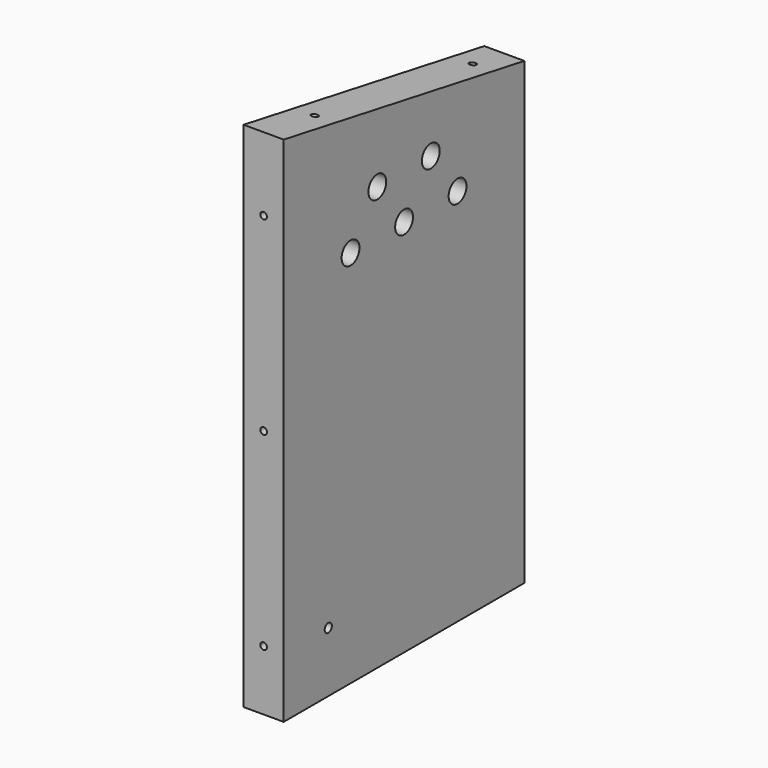
from build123d import *

# Parameters (mm, degrees)
F1_DEPTH       = 18
F2_D           = 10
F3_D           = 10
F4_D           = 4
F4_CSINK_D     = 8.2
F4_CSINK_ANGLE = 90
F6_D           = 3
F6_DEPTH       = 20
F6_TIP         = 0.9012909285
F8_D           = 3
F8_DEPTH       = 20
F8_TIP         = 0.9012909285
F10_D          = 3
F10_DEPTH      = 20
F10_TIP        = 0.9012909285


# Not quite as in the source:
# - a feature names something its author has since deleted; it is built from what else it names


with BuildPart() as f1:
    # F0 (on Right) → F1 (new body)
    with BuildSketch(Plane.YZ):
        Polygon((0, 230), (0, 0), (135, 0), (135, 206.1958576044), align=None)
    extrude(amount=F1_DEPTH)

    # F2 (through all)
    with Locations(Plane(origin=(0, 0, 0), x_dir=(0, 1, 0), z_dir=(-1, 0, 0))):
        with Locations((37.5, -170), (67.5, -170), (97.5, -170)):
            Hole(F2_D / 2)

    # F3 (through all)
    with Locations(Plane(origin=(0, 0, 0), x_dir=(0, 1, 0), z_dir=(-1, 0, 0))):
        with Locations((52.5, -190), (82.5, -190)):
            Hole(F3_D / 2)

    # F4 (through all)
    with Locations(Plane(origin=(0, 0, 0), x_dir=(0, 1, 0), z_dir=(-1, 0, 0))):
        with Locations((25, -27)):
            CounterSinkHole(F4_D / 2, F4_CSINK_D / 2, counter_sink_angle=F4_CSINK_ANGLE)

    # F6
    with Locations(Plane(origin=(0, 135, 0), x_dir=(-1, 0, 0), z_dir=(0, 1, 0))):
        with Locations((-9, 27), (-9, 106)):
            Hole(F6_D / 2, depth=F6_DEPTH)
            with Locations((0, 0, -(F6_DEPTH + F6_TIP / 2))):  # 118° drill point
                Cone(0, F6_D / 2, F6_TIP, mode=Mode.SUBTRACT)

    # F8
    with Locations(Plane.XZ):
        with Locations((9, 27), (9, 112), (9, 197)):
            Hole(F8_D / 2, depth=F8_DEPTH)
            with Locations((0, 0, -(F8_DEPTH + F8_TIP / 2))):  # 118° drill point
                Cone(0, F8_D / 2, F8_TIP, mode=Mode.SUBTRACT)

    # F10
    with Locations(Plane(origin=(0, 39.3323164825, 223.0646513904), x_dir=(1, 0, 0), z_dir=(0, 0.1736481777, 0.984807753))):
        with Locations((9, -10.8564882588), (9, 79.1435117412)):
            Hole(F10_D / 2, depth=F10_DEPTH)
            with Locations((0, 0, -(F10_DEPTH + F10_TIP / 2))):  # 118° drill point
                Cone(0, F10_D / 2, F10_TIP, mode=Mode.SUBTRACT)


solid = f1.part
